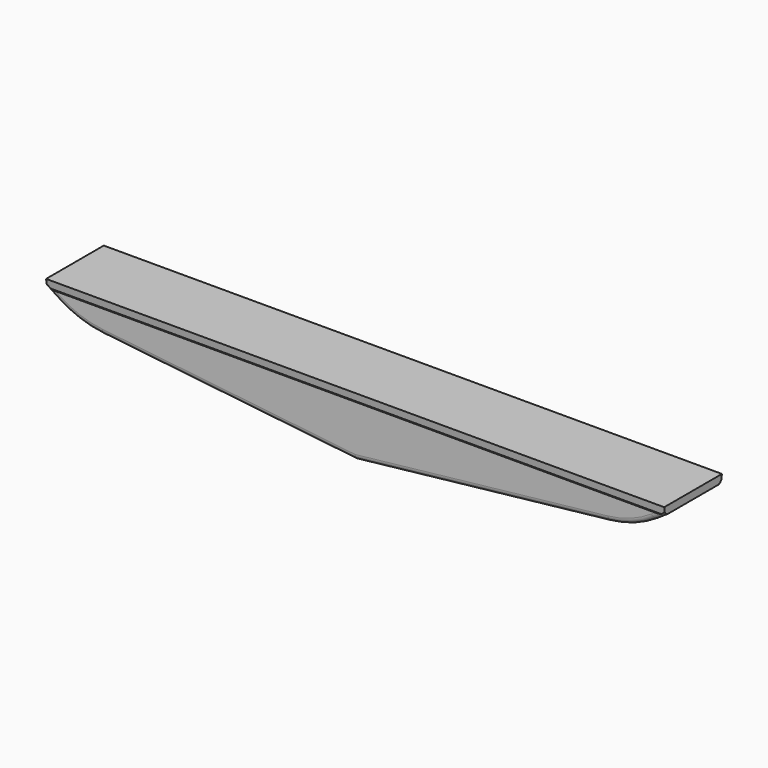
from build123d import *

# Parameters (mm, degrees)
F0_W          = 762
F0_H          = 9.525
F1_DEPTH      = 44.45
F2_W          = 31.75
F2_H          = 31.75
F3_DEPTH      = 25.4
F4_W          = 31.75
F4_H          = 31.75
F5_DEPTH      = 25.4
F7_DEPTH      = 762.001
F9_DEPTH      = 762.001
F10_T1_DEPTH  = 361.7347577498
F10_T3_DEPTH  = 361.7347577498
F10_T5_DEPTH  = 30.7650851852
F10_T7_DEPTH  = 30.7650851852
F10_T10_ANGLE = 27.3498757801
F10_T12_ANGLE = 27.3498757801
F10_T14_ANGLE = 27.3498757801
F10_T16_ANGLE = 27.3498757801


# Not quite as in the source:
# - a fillet or chamfer that OpenCascade refuses, or shapes differently, is made with other operations: its cross-section is extruded or revolved along the edge and cut away or added
# - a feature names something its author has since deleted; it is built from what else it names


with BuildPart() as f1:
    # F0 (on Front) → F1 (new body, symmetric)
    with BuildSketch(Plane.XZ):
        with Locations((0.726044178, 113.6916989031)):
            Rectangle(F0_W, F0_H)
        with BuildLine():
            Line((381.726044178, 108.9291989031), (-380.273955822, 108.9291989031))
            Line((-380.273955822, 108.9291989031), (-367.8846560609, 100.669665729))
            ThreePointArc((-367.8846560609, 100.669665729), (-340.9058012367, 87.0105643735), (-311.4625349518, 80.1168188064))
            Line((-311.4625349518, 80.1168188064), (0.726044178, 45.4291989031))
            Line((0.726044178, 45.4291989031), (31.5534211464, 48.8544630107))
            Line((31.5534211464, 48.8544630107), (312.9146233078, 80.1168188064))
            ThreePointArc((312.9146233078, 80.1168188064), (342.3578895927, 87.0105643735), (369.3367444169, 100.669665729))
            Line((369.3367444169, 100.669665729), (381.726044178, 108.9291989031))
        make_face()
    extrude(amount=F1_DEPTH, both=True)

    # F2 (on face) → F3 (cut)
    with BuildSketch(Plane(origin=(4.9949857842, 0, 44.954872058), x_dir=(0.9938837347, 0, -0.1104315261), z_dir=(-0.1104315261, 0, -0.9938837347))):
        with Locations((-32.870212264, 0)):
            Rectangle(F2_W, F2_H)
    extrude(amount=-F3_DEPTH, mode=Mode.SUBTRACT)

    # F4 (on face) → F5 (cut)
    with BuildSketch(Plane(origin=(-4.9772773896, 0, 44.7954965067), x_dir=(0.9938837347, 0, 0.1104315261), z_dir=(0.1104315261, 0, -0.9938837347))):
        with Locations((34.3134192624, 0)):
            Rectangle(F4_W, F4_H)
    extrude(amount=-F5_DEPTH, mode=Mode.SUBTRACT)

    # F6 (on face) → F7 (cut, through all)
    with BuildSketch(Plane.YZ.offset(381.726044178)):
        Polygon((-43.1113485495, 108.9291989031), (-44.45, 118.4541989031), (-44.45, 108.9291989031), align=None)
    extrude(amount=-F7_DEPTH, mode=Mode.SUBTRACT)

    # F8 (on face) → F9 (cut, through all)
    with BuildSketch(Plane.YZ.offset(381.726044178)):
        Polygon((44.45, 108.9291989031), (44.45, 118.4541989031), (43.1113485495, 108.9291989031), align=None)
    extrude(amount=-F9_DEPTH, mode=Mode.SUBTRACT)

    # F10: fillet of radius 6.35 on 4 edges, made by hand

    # F10_s2 → F10_t1 (cut)
    with BuildSketch(Plane(origin=(-316.457520736, 0, 35.1619467484), x_dir=(0, 1, 0), z_dir=(0.9938837347, 0, -0.1104315261))):
        with BuildLine():
            ThreePointArc((-44.45, 51.5815200356), (-42.5901280605, 47.0913919751), (-38.1, 45.2315200356))
            Line((-38.1, 45.2315200356), (-44.45, 45.2315200356))
            Line((-44.45, 45.2315200356), (-44.45, 51.5815200356))
        make_face()
        with BuildLine():
            ThreePointArc((44.45, 51.5815200356), (42.5901280605, 47.0913919751), (38.1, 45.2315200356))
            Line((38.1, 45.2315200356), (44.45, 45.2315200356))
            Line((44.45, 45.2315200356), (44.45, 51.5815200356))
        make_face()
    extrude(amount=F10_T1_DEPTH, mode=Mode.SUBTRACT)

    # F10_s4 → F10_t3 (cut)
    with BuildSketch(Plane(origin=(-41.6303912962, 0, -4.6255990329), x_dir=(0, 1, 0), z_dir=(0.9938837347, 0, 0.1104315261))):
        with BuildLine():
            ThreePointArc((-44.45, 51.4211637025), (-42.5901280605, 46.9310356419), (-38.1, 45.0711637025))
            Line((-38.1, 45.0711637025), (-44.45, 45.0711637025))
            Line((-44.45, 45.0711637025), (-44.45, 51.4211637025))
        make_face()
        with BuildLine():
            ThreePointArc((44.45, 51.4211637025), (42.5901280605, 46.9310356419), (38.1, 45.0711637025))
            Line((38.1, 45.0711637025), (44.45, 45.0711637025))
            Line((44.45, 45.0711637025), (44.45, 51.4211637025))
        make_face()
    extrude(amount=F10_T3_DEPTH, mode=Mode.SUBTRACT)

    # F10_s6 → F10_t5 (cut)
    with BuildSketch(Plane(origin=(-326.7503981008, 0, 217.8335987339), x_dir=(0, 1, 0), z_dir=(0.8320502943, 0, -0.5547001962))):
        with BuildLine():
            ThreePointArc((38.1, -120.3034659045), (42.5901280605, -118.443593965), (44.45, -113.9534659045))
            Line((44.45, -113.9534659045), (44.45, -120.3034659045))
            Line((44.45, -120.3034659045), (38.1, -120.3034659045))
        make_face()
        with BuildLine():
            ThreePointArc((-38.1, -120.3034659045), (-42.5901280605, -118.443593965), (-44.45, -113.9534659045))
            Line((-44.45, -113.9534659045), (-44.45, -120.3034659045))
            Line((-44.45, -120.3034659045), (-38.1, -120.3034659045))
        make_face()
    extrude(amount=F10_T5_DEPTH, mode=Mode.SUBTRACT)

    # F10_s8 → F10_t7 (cut)
    with BuildSketch(Plane(origin=(302.1575918559, 0, 201.4383945706), x_dir=(0, 1, 0), z_dir=(0.8320502943, 0, 0.5547001962))):
        with BuildLine():
            ThreePointArc((44.45, -114.7589396005), (42.5901280605, -119.2490676611), (38.1, -121.1089396005))
            Line((38.1, -121.1089396005), (44.45, -121.1089396005))
            Line((44.45, -121.1089396005), (44.45, -114.7589396005))
        make_face()
        with BuildLine():
            ThreePointArc((-44.45, -114.7589396005), (-42.5901280605, -119.2490676611), (-38.1, -121.1089396005))
            Line((-38.1, -121.1089396005), (-44.45, -121.1089396005))
            Line((-44.45, -121.1089396005), (-44.45, -114.7589396005))
        make_face()
    extrude(amount=F10_T7_DEPTH, mode=Mode.SUBTRACT)

    # F10_s9 → F10_t10 (revolve, cut)
    with BuildSketch(Plane(origin=(-301.1522999171, 0, 200.7681999448), x_dir=(0, 1, 0), z_dir=(-0.8320502943, 0, 0.5547001962))):
        with BuildLine():
            ThreePointArc((44.45, 113.9534659045), (42.5901280605, 118.443593965), (38.1, 120.3034659045))
            Line((38.1, 120.3034659045), (44.45, 120.3034659045))
            Line((44.45, 120.3034659045), (44.45, 113.9534659045))
        make_face()
    revolve(axis=Axis((-297.4377311403, 44.45, 206.34005311), (0, -1, 0)), revolution_arc=F10_T10_ANGLE, mode=Mode.SUBTRACT)

    # F10_s11 → F10_t12 (revolve, cut)
    with BuildSketch(Plane(origin=(317.8919006975, 0, 35.3213222997), x_dir=(0, 1, 0), z_dir=(-0.9938837347, 0, -0.1104315261))):
        with BuildLine():
            ThreePointArc((44.45, -51.4211637025), (42.5901280605, -46.9310356419), (38.1, -45.0711637025))
            Line((38.1, -45.0711637025), (44.45, -45.0711637025))
            Line((44.45, -45.0711637025), (44.45, -51.4211637025))
        make_face()
    revolve(axis=Axis((298.8898194963, 44.45, 206.34005311), (0, -1, 0)), revolution_arc=F10_T12_ANGLE, mode=Mode.SUBTRACT)

    # F10_s13 → F10_t14 (revolve, cut)
    with BuildSketch(Plane(origin=(317.8919006975, 0, 35.3213222997), x_dir=(0, 1, 0), z_dir=(-0.9938837347, 0, -0.1104315261))):
        with BuildLine():
            ThreePointArc((-44.45, -51.4211637025), (-42.5901280605, -46.9310356419), (-38.1, -45.0711637025))
            Line((-38.1, -45.0711637025), (-44.45, -45.0711637025))
            Line((-44.45, -45.0711637025), (-44.45, -51.4211637025))
        make_face()
    revolve(axis=Axis((298.8898194963, -44.45, 206.34005311), (0, -1, 0)), revolution_arc=F10_T14_ANGLE, mode=Mode.SUBTRACT)

    # F10_s15 → F10_t16 (revolve, cut)
    with BuildSketch(Plane(origin=(-301.1522999171, 0, 200.7681999448), x_dir=(0, 1, 0), z_dir=(-0.8320502943, 0, 0.5547001962))):
        with BuildLine():
            ThreePointArc((-38.1, 120.3034659045), (-42.5901280605, 118.443593965), (-44.45, 113.9534659045))
            Line((-44.45, 113.9534659045), (-44.45, 120.3034659045))
            Line((-44.45, 120.3034659045), (-38.1, 120.3034659045))
        make_face()
    revolve(axis=Axis((-297.4377311403, -44.45, 206.34005311), (0, -1, 0)), revolution_arc=F10_T16_ANGLE, mode=Mode.SUBTRACT)


solid = f1.part
